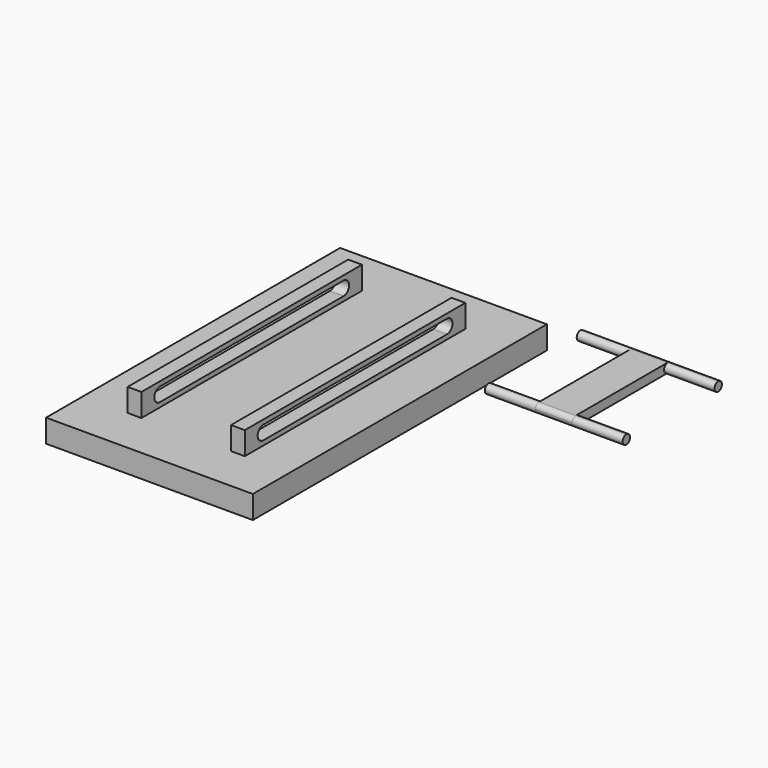
from build123d import *
from build123d import SkipClean  # not in build123d's __all__

# Parameters (mm, degrees)
F0_W      = 45
F0_H      = 80
F1_DEPTH  = 5
F2_W      = 3
F2_H      = 60
F3_DEPTH  = 5
F5_DEPTH  = 75.3
F6_W      = 8
F6_H      = 25
F7_DEPTH  = 2
F9_DEPTH  = 11
F11_DEPTH = 8
F10_R     = 1
F12_DEPTH = 11


with BuildPart() as f1:
    # F0 (on Top) → F1 (new body)
    with BuildSketch(Plane.XY):
        Rectangle(F0_W, F0_H)
    extrude(amount=F1_DEPTH)

    # F2 (on face) → F3 (join)
    with BuildSketch(Plane.XY.offset(5)):
        with Locations((-11.25, 0)):
            Rectangle(F2_W, F2_H)
        with Locations((11.25, 0)):
            Rectangle(F2_W, F2_H)
    extrude(amount=F3_DEPTH)

    # F4 (on face) → F5 (cut)
    with BuildSketch(Plane(origin=(-12.75, 0, 0), x_dir=(0, -1, 0), z_dir=(-1, 0, 0))):
        with BuildLine():
            ThreePointArc((-25, 6), (-23.9393398282, 6.4393398282), (-23.5, 7.5))
            ThreePointArc((-23.5, 7.5), (-23.9393398282, 8.5606601718), (-25, 9))
            ThreePointArc((-25, 9), (-26.5, 7.5), (-25, 6))
        make_face()
        with BuildLine():
            ThreePointArc((-25, 9), (-23.9393398282, 8.5606601718), (-23.5, 7.5))
            ThreePointArc((-23.5, 7.5), (-23.9393398282, 6.4393398282), (-25, 6))
            Line((-25, 6), (0, 6))
            Line((0, 6), (25, 6))
            ThreePointArc((25, 6), (23.5, 7.5), (25, 9))
            Line((25, 9), (0, 9))
            Line((0, 9), (-25, 9))
        make_face()
        with BuildLine():
            ThreePointArc((26.5, 7.5), (26.0606601718, 8.5606601718), (25, 9))
            ThreePointArc((25, 9), (23.5, 7.5), (25, 6))
            ThreePointArc((25, 6), (26.0606601718, 6.4393398282), (26.5, 7.5))
        make_face()
    extrude(amount=-F5_DEPTH, mode=Mode.SUBTRACT)


with BuildPart() as f7:
    # F6 (on Top) → F7 (new body)
    with BuildSketch(Plane.XY):
        with Locations((39.7293449342, 33.835914731)):
            Rectangle(F6_W, F6_H)
    extrude(amount=F7_DEPTH)

    # F8 (on face) → F9 (join)
    with BuildSketch(Plane.YZ.offset(43.7293449342)):
        with BuildLine():
            Line((21.335914731, 0), (21.335914731, 2))
            ThreePointArc((21.335914731, 2), (20.335914731, 1), (21.335914731, 0))
        make_face()
        with BuildLine():
            ThreePointArc((21.335914731, 0), (22.0430215122, 0.2928932188), (22.335914731, 1))
            ThreePointArc((22.335914731, 1), (22.0430215122, 1.7071067812), (21.335914731, 2))
            Line((21.335914731, 2), (21.335914731, 0))
        make_face()
        with BuildLine():
            Line((46.335914731, 0), (46.335914731, 2))
            ThreePointArc((46.335914731, 2), (45.335914731, 1), (46.335914731, 0))
        make_face()
        with BuildLine():
            ThreePointArc((47.335914731, 1), (47.0430215122, 1.7071067812), (46.335914731, 2))
            Line((46.335914731, 2), (46.335914731, 0))
            ThreePointArc((46.335914731, 0), (47.0430215122, 0.2928932188), (47.335914731, 1))
        make_face()
    extrude(amount=F9_DEPTH)

    # F10 (on face) → F11 (join, through all)
    with BuildSketch(Plane(origin=(35.7293449342, 0, 0), x_dir=(0, -1, 0), z_dir=(-1, 0, 0))):
        with BuildLine():
            ThreePointArc((-21.335914731, 0), (-20.6288079498, 0.2928932188), (-20.335914731, 1))
            ThreePointArc((-20.335914731, 1), (-20.6288079498, 1.7071067812), (-21.335914731, 2))
            Line((-21.335914731, 2), (-21.335914731, 0))
        make_face()
        with BuildLine():
            Line((-21.335914731, 0), (-21.335914731, 2))
            ThreePointArc((-21.335914731, 2), (-22.335914731, 1), (-21.335914731, 0))
        make_face()
        with BuildLine():
            Line((-46.335914731, 0), (-46.335914731, 2))
            ThreePointArc((-46.335914731, 2), (-47.335914731, 1), (-46.335914731, 0))
        make_face()
        with BuildLine():
            ThreePointArc((-45.335914731, 1), (-45.6288079498, 1.7071067812), (-46.335914731, 2))
            Line((-46.335914731, 2), (-46.335914731, 0))
            ThreePointArc((-46.335914731, 0), (-45.6288079498, 0.2928932188), (-45.335914731, 1))
        make_face()
    with SkipClean():  # cleaning this boolean's faces spoils the solid; the shape is the same uncleaned
        extrude(amount=-F11_DEPTH)

    # F10 (on face) → F12 (join)
    with BuildSketch(Plane(origin=(35.7293449342, 0, 0), x_dir=(0, -1, 0), z_dir=(-1, 0, 0))):
        with Locations((-21.335914731, 1)):
            Circle(F10_R)
        with Locations((-46.335914731, 1)):
            Circle(F10_R)
    extrude(amount=F12_DEPTH)


solid = Compound([f1.part, f7.part])
